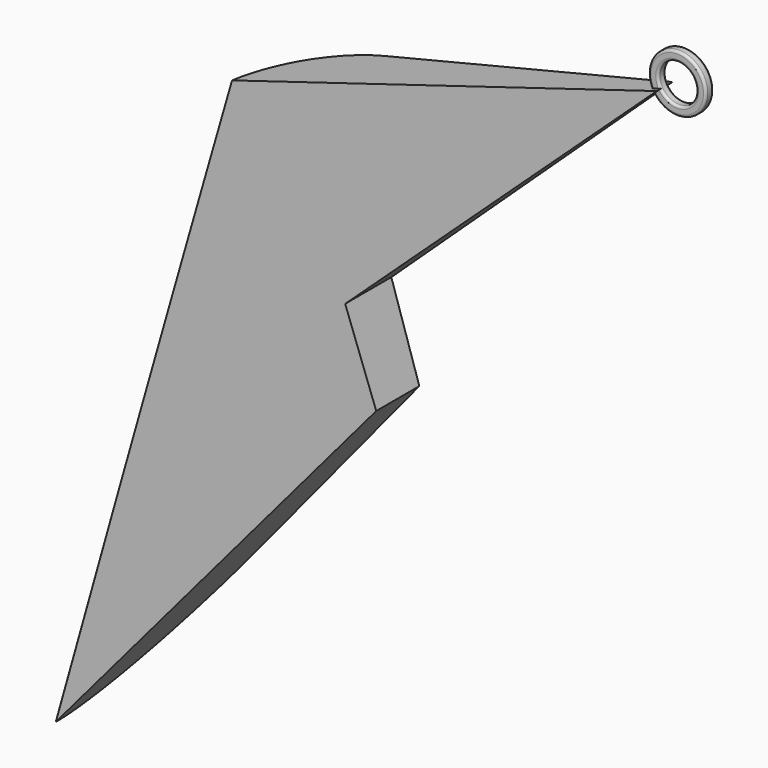
from build123d import *

# Parameters (mm, degrees)
F1_DEPTH      = 5
F1_DEPTH_BACK = 5
F2_W          = 100.360032171
F2_H          = 34.278569743
F3_DEPTH      = 63.9
F3_DEPTH_BACK = 50
F4_R          = 0.0218183936
F5_T1_DEPTH   = 111.9716351384
F6_R          = 3
F6_R_2        = 2
F7_DEPTH      = 0.5
F7_DEPTH_BACK = 0.5
F8_T4_ANGLE   = 359.64
F8_T9_ANGLE   = 359.64
F8_T34_ANGLE  = 359.64
F8_T39_ANGLE  = 359.64


# Not quite as in the source:
# - a fillet or chamfer that OpenCascade refuses, or shapes differently, is made with other operations: its cross-section is extruded or revolved along the edge and cut away or added


with BuildPart() as f1:
    # F0 (on Front) → F1 (new body, two sides)
    with BuildSketch(Plane.XZ) as f1_sk:
        Polygon((31.0921985656, 30.5286794901), (-11.5655744448, 18.7216177583), (-28.8952961564, -45.6459186971), (3.0980354641, -7.3681822978), (0, 1.582333236), align=None)
    extrude(amount=F1_DEPTH)
    extrude(f1_sk.sketch, amount=-F1_DEPTH_BACK)

    # F2 (on Top) → F3 (cut, two sides)
    with BuildSketch(Plane.XY) as f3_sk:
        with Locations((1.9043665379, 3.6182934418)):
            Rectangle(F2_W, F2_H)
        Polygon((-39.0896312892, -5.3307767957), (-39.0896312892, 5.7227437609), (47.1330322325, 0), align=None, mode=Mode.SUBTRACT)
    extrude(amount=-F3_DEPTH, mode=Mode.SUBTRACT)
    extrude(f3_sk.sketch, amount=F3_DEPTH_BACK, mode=Mode.SUBTRACT)

    # F4
    f4_edges = [f1.edges().sort_by_distance(p)[0] for p in [
        (-20.230435, -4.164794, -13.46215),
    ]]
    fillet(f4_edges, radius=F4_R)

    # F5: fillet of radius 9 on 2 edges, made by hand

    # F5_s2 → F5_t1 (cut)
    with BuildSketch(Plane(origin=(10.1347631785, -0.6726613442, 37.6434053136), x_dir=(-0.0662259794, -0.99780465, 0), z_dir=(-0.259934786, 0.0172523106, -0.9654720425))):
        with BuildLine():
            ThreePointArc((6.4541084226, 15.6543338505), (-0.2785467468, 13.2370471707), (-3.1214312203, 6.6727552521))
            Line((-3.1214312203, 6.6727552521), (-3.1214312203, 16.2679345229))
            Line((-3.1214312203, 16.2679345229), (6.4541084226, 15.6543338505))
        make_face()
    extrude(amount=F5_T1_DEPTH, mode=Mode.SUBTRACT)

    # F6 (on Front) → F7 (join, two sides)
    with BuildSketch(Plane.XZ) as f7_sk:
        with Locations((32.8437015414, 31.5673612058)):
            Circle(F6_R)
        with Locations((32.8437015414, 31.5673612058)):
            Circle(F6_R_2, mode=Mode.SUBTRACT)
    extrude(amount=F7_DEPTH)
    extrude(f7_sk.sketch, amount=-F7_DEPTH_BACK)

    # F8: fillet of radius 0.25 on 4 edges, made by hand


with BuildPart() as f8_tool2:
    # F8_s3 → F8_t4 (revolve)
    with BuildSketch(Plane(origin=(-5.375639349, 0, 9.1752631985), x_dir=(0, 1, 0), z_dir=(-0.5055120978, 0, 0.8628195171))):
        with BuildLine():
            ThreePointArc((0.25, -41.2958696863), (0.4267766953, -41.369092991), (0.5, -41.5458696863))
            Line((0.5, -41.5458696863), (0.5, -41.2958696863))
            Line((0.5, -41.2958696863), (0.25, -41.2958696863))
        make_face()
    revolve(axis=Axis((32.8437015414, 0.5, 31.5673612058), (0, -1, 0)), revolution_arc=F8_T4_ANGLE)

    split(bisect_by=Plane(origin=(-0.7891478665, 0, 0.8476490244), x_dir=(0, 1, 0), z_dir=(0.6813988218, 0, -0.731912321)), keep=Keep.TOP)


with BuildPart() as f1_1:
    add(f1.part)

    # F8_t1: cut F8_tool2
    add(f8_tool2.part, mode=Mode.SUBTRACT)


with BuildPart() as f8_tool7:
    # F8_s8 → F8_t9 (revolve)
    with BuildSketch(Plane(origin=(-5.375639349, 0, 9.1752631985), x_dir=(0, 1, 0), z_dir=(-0.5055120978, 0, 0.8628195171))):
        with BuildLine():
            ThreePointArc((0.25, -41.2958696863), (0.4267766953, -41.369092991), (0.5, -41.5458696863))
            Line((0.5, -41.5458696863), (0.5, -41.2958696863))
            Line((0.5, -41.2958696863), (0.25, -41.2958696863))
        make_face()
    revolve(axis=Axis((32.8437015414, 0.5, 31.5673612058), (0, -1, 0)), revolution_arc=F8_T9_ANGLE)

    split(bisect_by=Plane(origin=(-5.636132621, 0, 20.3628024875), x_dir=(0, 1, 0), z_dir=(-0.2667561154, 0, 0.963764066)), keep=Keep.TOP)


with BuildPart() as f1_2:
    add(f1_1.part)

    # F8_t6: cut F8_tool7
    add(f8_tool7.part, mode=Mode.SUBTRACT)


with BuildPart() as f8_tool12:
    # F8_s13 → F8_t14 (revolve)
    with BuildSketch(Plane.XY.offset(31.5673612058)):
        with BuildLine():
            ThreePointArc((35.0937015414, -0.5), (34.9169248461, -0.4267766953), (34.8437015414, -0.25))
            Line((34.8437015414, -0.25), (34.8437015414, -0.5))
            Line((34.8437015414, -0.5), (35.0937015414, -0.5))
        make_face()
    revolve(axis=Axis((32.8437015414, -0.5, 31.5673612058), (0, -1, 0)))

    split(bisect_by=Plane(origin=(-0.7891478665, 0, 0.8476490244), x_dir=(0, 1, 0), z_dir=(0.6813988218, 0, -0.731912321)), keep=Keep.TOP)


with BuildPart() as f1_3:
    add(f1_2.part)

    # F8_t11: cut F8_tool12
    add(f8_tool12.part, mode=Mode.SUBTRACT)


with BuildPart() as f8_tool17:
    # F8_s18 → F8_t19 (revolve)
    with BuildSketch(Plane.XY.offset(31.5673612058)):
        with BuildLine():
            ThreePointArc((35.0937015414, -0.5), (34.9169248461, -0.4267766953), (34.8437015414, -0.25))
            Line((34.8437015414, -0.25), (34.8437015414, -0.5))
            Line((34.8437015414, -0.5), (35.0937015414, -0.5))
        make_face()
    revolve(axis=Axis((32.8437015414, -0.5, 31.5673612058), (0, -1, 0)))

    split(bisect_by=Plane(origin=(-5.636132621, 0, 20.3628024875), x_dir=(0, 1, 0), z_dir=(-0.2667561154, 0, 0.963764066)), keep=Keep.TOP)


with BuildPart() as f1_4:
    add(f1_3.part)

    # F8_t16: cut F8_tool17
    add(f8_tool17.part, mode=Mode.SUBTRACT)


with BuildPart() as f8_tool22:
    # F8_s23 → F8_t24 (revolve)
    with BuildSketch(Plane.XY.offset(31.5673612058)):
        with BuildLine():
            ThreePointArc((34.8437015414, 0.25), (34.9169248461, 0.4267766953), (35.0937015414, 0.5))
            Line((35.0937015414, 0.5), (34.8437015414, 0.5))
            Line((34.8437015414, 0.5), (34.8437015414, 0.25))
        make_face()
    revolve(axis=Axis((32.8437015414, 0.5, 31.5673612058), (0, -1, 0)))

    split(bisect_by=Plane(origin=(-0.7891478665, 0, 0.8476490244), x_dir=(0, 1, 0), z_dir=(0.6813988218, 0, -0.731912321)), keep=Keep.TOP)


with BuildPart() as f1_5:
    add(f1_4.part)

    # F8_t21: cut F8_tool22
    add(f8_tool22.part, mode=Mode.SUBTRACT)


with BuildPart() as f8_tool27:
    # F8_s28 → F8_t29 (revolve)
    with BuildSketch(Plane.XY.offset(31.5673612058)):
        with BuildLine():
            ThreePointArc((34.8437015414, 0.25), (34.9169248461, 0.4267766953), (35.0937015414, 0.5))
            Line((35.0937015414, 0.5), (34.8437015414, 0.5))
            Line((34.8437015414, 0.5), (34.8437015414, 0.25))
        make_face()
    revolve(axis=Axis((32.8437015414, 0.5, 31.5673612058), (0, -1, 0)))

    split(bisect_by=Plane(origin=(-5.636132621, 0, 20.3628024875), x_dir=(0, 1, 0), z_dir=(-0.2667561154, 0, 0.963764066)), keep=Keep.TOP)


with BuildPart() as f1_6:
    add(f1_5.part)

    # F8_t26: cut F8_tool27
    add(f8_tool27.part, mode=Mode.SUBTRACT)


with BuildPart() as f8_tool32:
    # F8_s33 → F8_t34 (revolve)
    with BuildSketch(Plane(origin=(-5.375639349, 0, 9.1752631985), x_dir=(0, 1, 0), z_dir=(-0.5055120978, 0, 0.8628195171))):
        with BuildLine():
            ThreePointArc((-0.5, -41.5458696863), (-0.4267766953, -41.369092991), (-0.25, -41.2958696863))
            Line((-0.25, -41.2958696863), (-0.5, -41.2958696863))
            Line((-0.5, -41.2958696863), (-0.5, -41.5458696863))
        make_face()
    revolve(axis=Axis((32.8437015414, -0.5, 31.5673612058), (0, -1, 0)), revolution_arc=F8_T34_ANGLE)

    split(bisect_by=Plane(origin=(-0.7891478665, 0, 0.8476490244), x_dir=(0, 1, 0), z_dir=(0.6813988218, 0, -0.731912321)), keep=Keep.TOP)


with BuildPart() as f1_7:
    add(f1_6.part)

    # F8_t31: cut F8_tool32
    add(f8_tool32.part, mode=Mode.SUBTRACT)


with BuildPart() as f8_tool37:
    # F8_s38 → F8_t39 (revolve)
    with BuildSketch(Plane(origin=(-5.375639349, 0, 9.1752631985), x_dir=(0, 1, 0), z_dir=(-0.5055120978, 0, 0.8628195171))):
        with BuildLine():
            ThreePointArc((-0.5, -41.5458696863), (-0.4267766953, -41.369092991), (-0.25, -41.2958696863))
            Line((-0.25, -41.2958696863), (-0.5, -41.2958696863))
            Line((-0.5, -41.2958696863), (-0.5, -41.5458696863))
        make_face()
    revolve(axis=Axis((32.8437015414, -0.5, 31.5673612058), (0, -1, 0)), revolution_arc=F8_T39_ANGLE)

    split(bisect_by=Plane(origin=(-5.636132621, 0, 20.3628024875), x_dir=(0, 1, 0), z_dir=(-0.2667561154, 0, 0.963764066)), keep=Keep.TOP)


with BuildPart() as f1_8:
    add(f1_7.part)

    # F8_t36: cut F8_tool37
    add(f8_tool37.part, mode=Mode.SUBTRACT)


solid = f1_8.part
